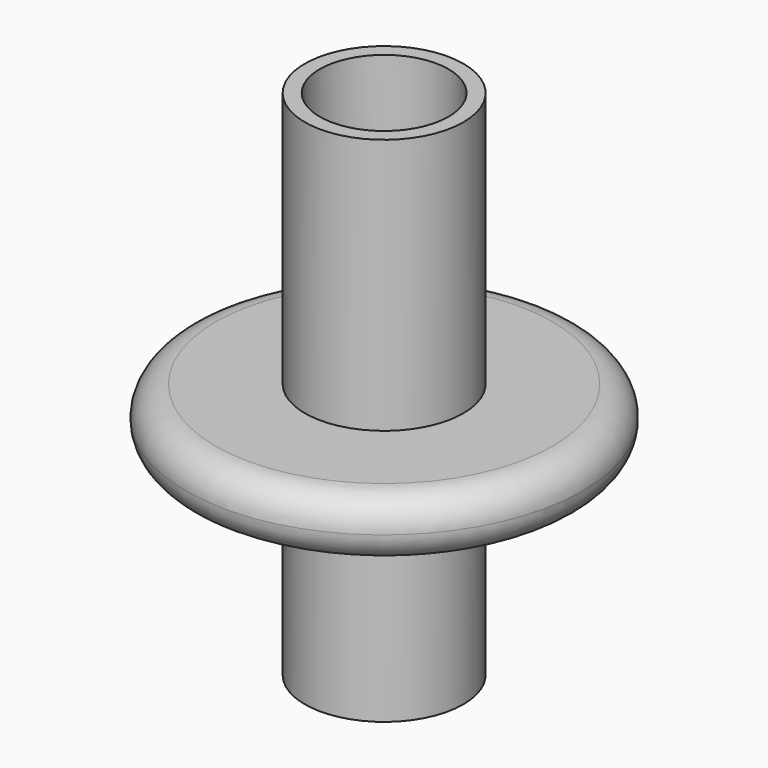
from build123d import *

# Parameters (mm, degrees)
F0_R           = 100
F1_DEPTH       = 30
F2_R           = 40
F3_DEPTH       = 129.3
F4_R           = 14.99999
F6_D           = 45
F6_DEPTH       = 200
F6_CBORE_D     = 65
F6_CBORE_DEPTH = 80
F6_TIP         = 13.5193639281


# Not quite as in the source:
# - a fillet or chamfer is up to 0.001 mm smaller than in the source, because OpenCascade refuses the exact size


with BuildPart() as f1:
    # F0 (on Top) → F1 (new body)
    with BuildSketch(Plane.XY):
        Circle(F0_R)
    extrude(amount=F1_DEPTH)

    # F2 (on face) → F3 (join, symmetric)
    with BuildSketch(Plane.XY.offset(30)):
        Circle(F2_R)
    extrude(amount=F3_DEPTH, both=True)

    # F4 (radius 15 in the source; OpenCascade refuses exactly that, so slightly less here)
    f4_edges = [f1.edges().sort_by_distance(p)[0] for p in [
        (-100, 0, 30),
        (100, 0, 15),
        (-100, 0, 0),
    ]]
    fillet(f4_edges, radius=F4_R)

    # F6
    with Locations(Plane.XY.offset(159.3)):
        with Locations((0, 0)):
            CounterBoreHole(F6_D / 2, F6_CBORE_D / 2, F6_CBORE_DEPTH, depth=F6_DEPTH)
            with Locations((0, 0, -(F6_DEPTH + F6_TIP / 2))):  # 118° drill point
                Cone(0, F6_D / 2, F6_TIP, mode=Mode.SUBTRACT)


solid = f1.part
